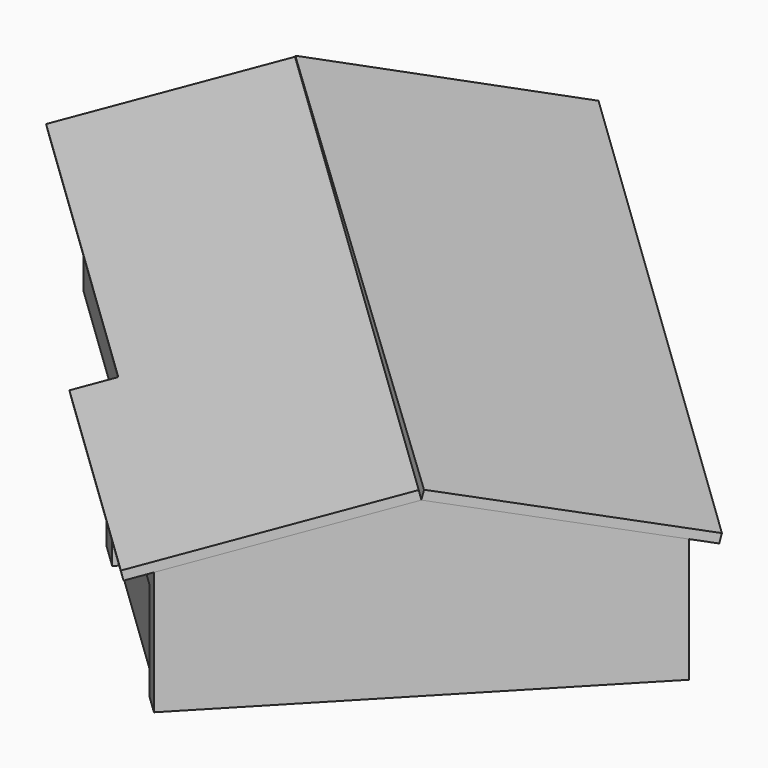
from build123d import *

# Parameters (mm, degrees)
F1_DEPTH  = 4267.2
F3_DEPTH  = 22404.0093298425
F4_W      = 5486.4
F4_H      = 2438.4
F5_DEPTH  = 152.4
F6_W      = 1066.8
F6_H      = 2438.4
F6_W_2    = 1524
F6_H_2    = 1524
F6_W_3    = 1360.4601135254
F6_H_3    = 1063.0166530609
F7_DEPTH  = 100.584
F9_DEPTH  = 228.6
F11_DEPTH = 228.6


with BuildPart() as f1:
    # F0 (on Top) → F1 (new body)
    with BuildSketch(Plane.XY):
        Polygon((22143.9891962815, -28323.0176376037), (9394.0277099609, -16083.0516815186), (2837.5189186279, -22912.7467047027), (10540.6964407008, -30307.7988956456), (9880.2969050223, -30995.7149140147), (14927.08086927, -35840.628679157), align=None)
    extrude(amount=F1_DEPTH)

    # F2 (on face) → F3 (cut, through all)
    with BuildSketch(Plane(origin=(25673.4394830699, -24646.5078020462, 0), x_dir=(0.6925319144, 0.7213872382, 0), z_dir=(0.7213872382, -0.6925319144, 0))):
        Polygon((-5096.4442406311, 4267.2), (-10306.968244332, 4267.2), (-5025.367095683, 3048), align=None)
        Polygon((-10306.968244332, 4267.2), (-15517.4922480328, 4267.2), (-15517.4922480328, 3048), align=None)
    extrude(amount=-F3_DEPTH, mode=Mode.SUBTRACT)

    # F4 (on face) → F5 (cut)
    with BuildSketch(Plane(origin=(-10746.3586137999, -11194.1208771108, 0), x_dir=(0.7213872382, -0.6925319144, 0), z_dir=(-0.6925319144, -0.7213872382, 0))):
        with Locations((32159.9848369854, 1219.2)):
            Rectangle(F4_W, F4_H)
    extrude(amount=-F5_DEPTH, mode=Mode.SUBTRACT)

    # F6 (on face) → F7 (cut)
    with BuildSketch(Plane(origin=(-10085.9590781215, -10506.2048587416, 0), x_dir=(0.7213872382, -0.6925319144, 0), z_dir=(-0.6925319144, -0.7213872382, 0))):
        with Locations((27426.589012146, 1524)):
            Rectangle(F6_W, F6_H)
        with Locations((24917.7712554932, 1984.513794899)):
            Rectangle(F6_W_2, F6_H_2)
        with Locations((19561.8027801514, 2101.5466451645)):
            Rectangle(F6_W_3, F6_H_3)
    extrude(amount=-F7_DEPTH, mode=Mode.SUBTRACT)

    # F8 (on face) → F9 (join)
    with BuildSketch(Plane(origin=(-1026.0984542937, -1068.8523007626, 6332.2155253973), x_dir=(0.9874739089, -0.0262615306, 0.155581526), z_dir=(-0.1577823793, -0.1643566058, 0.9736999676))):
        Polygon((10851.9047445382, -29369.6509092254), (10183.1280510822, -30085.1097214559), (15739.266370424, -35278.7221979155), (19809.7725017939, -30924.0855749234), (6452.7419740348, -18438.5720023167), (3051.0125361209, -22077.7498130783), align=None)
    extrude(amount=F9_DEPTH)

    # F10 (on face) → F11 (join)
    with BuildSketch(Plane(origin=(286.5449578876, 298.4842597009, 1792.4358695192), x_dir=(0.9877938033, -0.0255866872, -0.1536513049), z_dir=(0.1557671406, 0.1622573992, 0.9743762796))):
        Polygon((5052.9201327622, -19930.4707746463), (18474.4933741329, -32346.9859386226), (22543.9703278489, -27996.4721098459), (9220.0241803924, -15533.2335330653), align=None)
    extrude(amount=F11_DEPTH)


solid = f1.part
